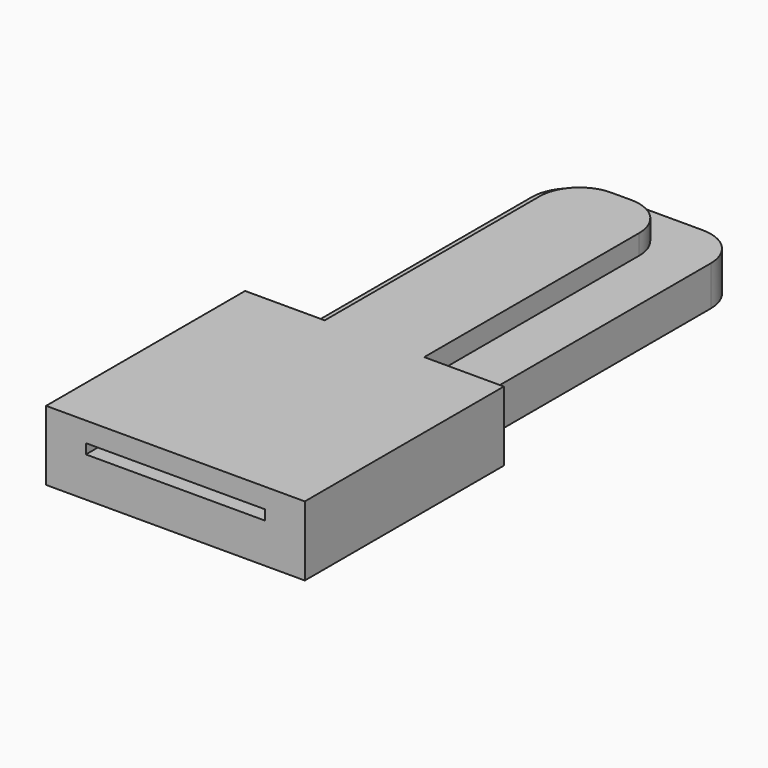
from build123d import *

# Parameters (mm, degrees)
F0_W     = 2
F0_H     = 10
F0_W_2   = 9
F0_H_2   = 2.5
F0_H_3   = 15
F1_DEPTH = 2
F2_DEPTH = 0.5
F3_W     = 2
F3_H     = 10
F3_W_2   = 5
F3_H_2   = 15.5
F4_DEPTH = 1
F5_R     = 2
F6_DEPTH = 25
F7_DEPTH = 2.5


# Not quite as in the source:
# - a feature names something its author has since deleted; it is built from what else it names


with BuildPart() as f1:
    # F0 (on Top) → F1 (new body)
    with BuildSketch(Plane.XY):
        with Locations((-5.5, -7.5)):
            Rectangle(F0_W, F0_H)
        with Locations((0, 13.75)):
            Rectangle(F0_W_2, F0_H_2)
        Polygon((4.5, -2.5), (4.5, 12.5), (-4.5, 12.5), (-4.5, -2.5), (-4.5, -12.5), (4.5, -12.5), align=None)
        with Locations((0, -13.75)):
            Rectangle(F0_W_2, F0_H_2)
        with Locations((5.5, -7.5)):
            Rectangle(F0_W, F0_H)
        with Locations((-5.5, 5)):
            Rectangle(F0_W, F0_H_3)
        with Locations((5.5, 5)):
            Rectangle(F0_W, F0_H_3)
    extrude(amount=-F1_DEPTH)

    # F0 (on Top) → F2 (join)
    with BuildSketch(Plane.XY):
        with Locations((-5.5, -7.5)):
            Rectangle(F0_W, F0_H)
        with Locations((5.5, -7.5)):
            Rectangle(F0_W, F0_H)
    extrude(amount=F2_DEPTH)

    # F3 (on face) → F4 (join)
    with BuildSketch(Plane.XY.offset(0.5)):
        with Locations((-5.5, -7.5)):
            Rectangle(F3_W, F3_H)
        Polygon((-4.5, -2.5), (-4.5, -12.5), (6.5, -12.5), (6.5, -2.5), (4.5, -2.5), (2.5, -2.5), (-2.5, -2.5), align=None)
        with Locations((0, 5.25)):
            Rectangle(F3_W_2, F3_H_2)
    extrude(amount=F4_DEPTH)

    # F5
    f5_edges = [f1.edges().sort_by_distance(p)[0] for p in [
        (-4.5, 15, -1),
        (4.5, 15, -1),
        (-2.5, 13, 1),
        (2.5, 13, 1),
    ]]
    fillet(f5_edges, radius=F5_R)

    # F0 (on Top) → F6 (cut)
    with BuildSketch(Plane.XY):
        with Locations((-5.5, 5)):
            Rectangle(F0_W, F0_H_3)
        with Locations((5.5, 5)):
            Rectangle(F0_W, F0_H_3)
    extrude(amount=-F6_DEPTH, mode=Mode.SUBTRACT)

    # F7 (add, through all): a face of the model
    f7_faces = [f1.faces().sort_by_distance(p)[0] for p in [
        (-5.5, -12.5, -1.8653708798),
    ]]
    extrude(f7_faces, amount=F7_DEPTH)


solid = f1.part
